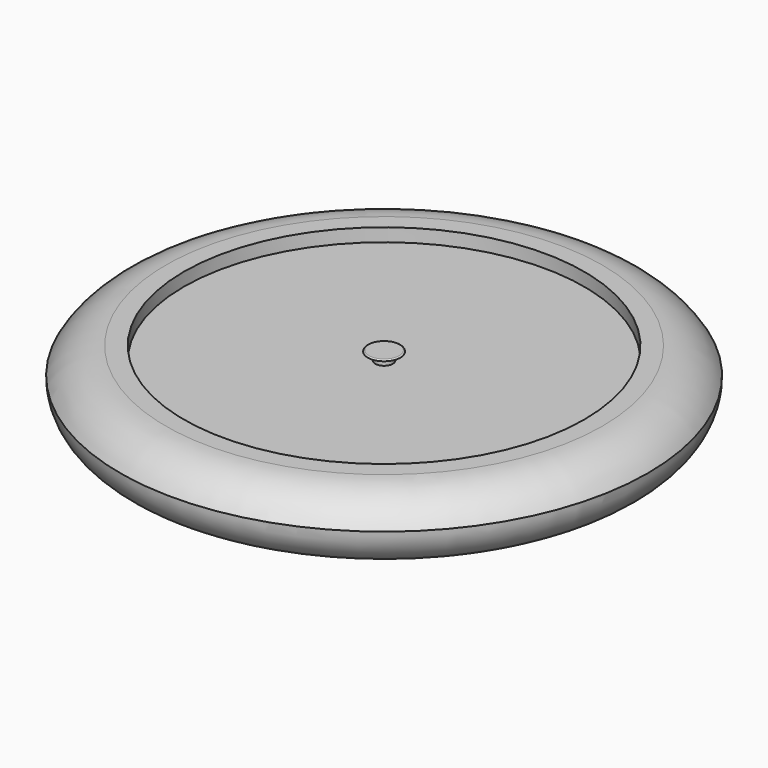
from build123d import *

# Parameters (mm, degrees)
F0_R     = 25.4
F1_DEPTH = 6.35
F2_R     = 3.81
F4_R     = 19.2670598269
F5_DEPTH = 1.27
F6_R     = 0.8432395902
F7_DEPTH = 0.762
F8_R     = 1.5748
F8_R_2   = 0.8432395902
F9_DEPTH = 0.127
F10_R    = 0.12699


# Not quite as in the source:
# - a fillet or chamfer that OpenCascade refuses, or shapes differently, is made with other operations: its cross-section is extruded or revolved along the edge and cut away or added
# - a fillet or chamfer is up to 0.001 mm smaller than in the source, because OpenCascade refuses the exact size


with BuildPart() as f1:
    # F0 (on Top) → F1 (new body)
    with BuildSketch(Plane.XY):
        Circle(F0_R)
    extrude(amount=F1_DEPTH)

    # F2
    f2_edges = [f1.edges().sort_by_distance(p)[0] for p in [
        (-25.4, 0, 0),
    ]]
    fillet(f2_edges, radius=F2_R)

    # F3: fillet of radius 5.08 on 1 edges, made by hand

    # F3_s1 → F3_t2 (revolve, cut)
    with BuildSketch(Plane.XZ):
        with BuildLine():
            ThreePointArc((25.4, 3.81), (23.5405909488, 5.6694090512), (21.0005909488, 6.35))
            Line((21.0005909488, 6.35), (25.4, 6.35))
            Line((25.4, 6.35), (25.4, 3.81))
        make_face()
    revolve(axis=Axis((0, 0, 6.35), (0, 0, 1)), mode=Mode.SUBTRACT)

    # F4 (on face) → F5 (cut)
    with BuildSketch(Plane.XY.offset(6.35)):
        Circle(F4_R)
    extrude(amount=-F5_DEPTH, mode=Mode.SUBTRACT)

    # F6 (on face) → F7 (join)
    with BuildSketch(Plane.XY.offset(5.08)):
        Circle(F6_R)
    extrude(amount=F7_DEPTH)

    # F8 (on face) → F9 (join)
    with BuildSketch(Plane.XY.offset(5.842)):
        Circle(F8_R)
        Circle(F8_R_2, mode=Mode.SUBTRACT)
        Circle(F8_R_2)
    extrude(amount=F9_DEPTH)

    # F10 (radius 0.127 in the source; OpenCascade refuses exactly that, so slightly less here)
    f10_edges = [f1.edges().sort_by_distance(p)[0] for p in [
        (-1.5748, 0, 5.969),
    ]]
    fillet(f10_edges, radius=F10_R)


solid = f1.part
